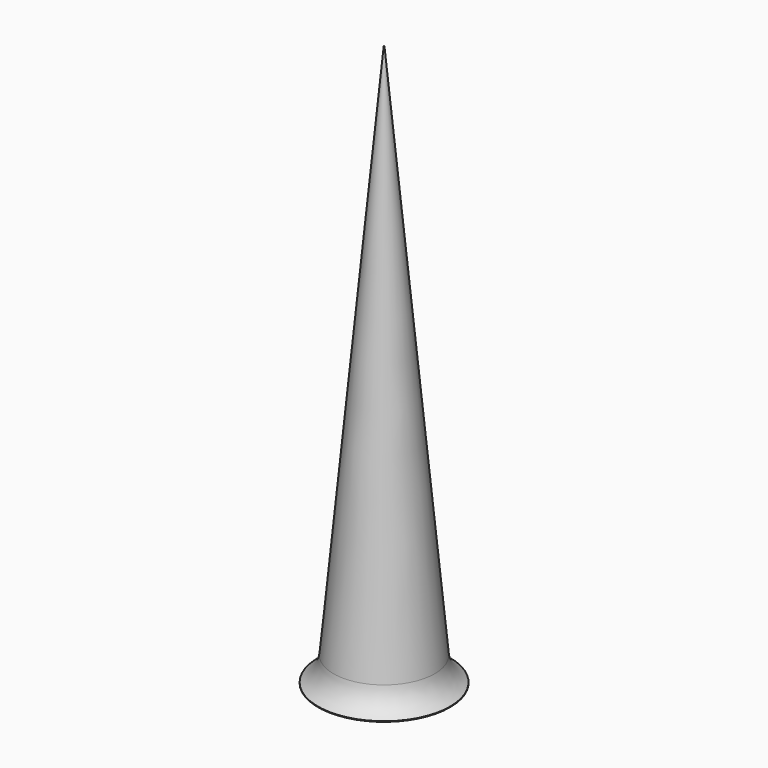
from build123d import *

# Parameters (mm, degrees)
F0_R     = 85
F2_R     = 0.5
F4_R     = 105.9677495378
F5_DEPTH = 1


# Not quite as in the source:
# - a fillet or chamfer that OpenCascade refuses, or shapes differently, is made with other operations: its cross-section is extruded or revolved along the edge and cut away or added


with BuildPart() as f3:
    # F0 (on Top) → F3 section 0
    with BuildSketch(Plane.XY):
        Circle(F0_R)
    # F2 (on offset) → F3 section 1
    with BuildSketch(Plane.XY.offset(900)):
        Circle(F2_R)
    loft()

    # F4 (on Top) → F5 (join)
    with BuildSketch(Plane.XY):
        Circle(F4_R)
    extrude(amount=F5_DEPTH)

    # F6: fillet of radius 50 on 1 edges, made by hand


with BuildPart() as f6_tool2:
    # F6_s3 → F6_t4 (revolve)
    with BuildSketch(Plane.XZ):
        with BuildLine():
            ThreePointArc((105.9675487491, 0.9996540464), (88.9507928559, 17.2936216176), (81.2843067656, 39.5711518076))
            Line((81.2843067656, 39.5711518076), (76.3060471064, 39.1037485396))
            ThreePointArc((76.3060471064, 39.1037485396), (78.1171484035, 19.8181913314), (79.927851452, 0.532596732))
            Line((79.927851452, 0.532596732), (84.9061111111, -4.0001535025))
            ThreePointArc((84.9061111111, -4.0001535025), (95.4368299301, -4.0001535025), (103.4576132883, -3.3248989977))
            Line((103.4576132883, -3.3248989977), (105.9675487491, 0.9996540464))
        make_face()
    revolve(axis=Axis((0, 0, 1), (0, 0, 1)))

    split(bisect_by=Plane.XY, keep=Keep.TOP)


with BuildPart() as f3_1:
    add(f3.part)

    # F6_t1: union F6_tool2
    add(f6_tool2.part)


solid = f3_1.part
